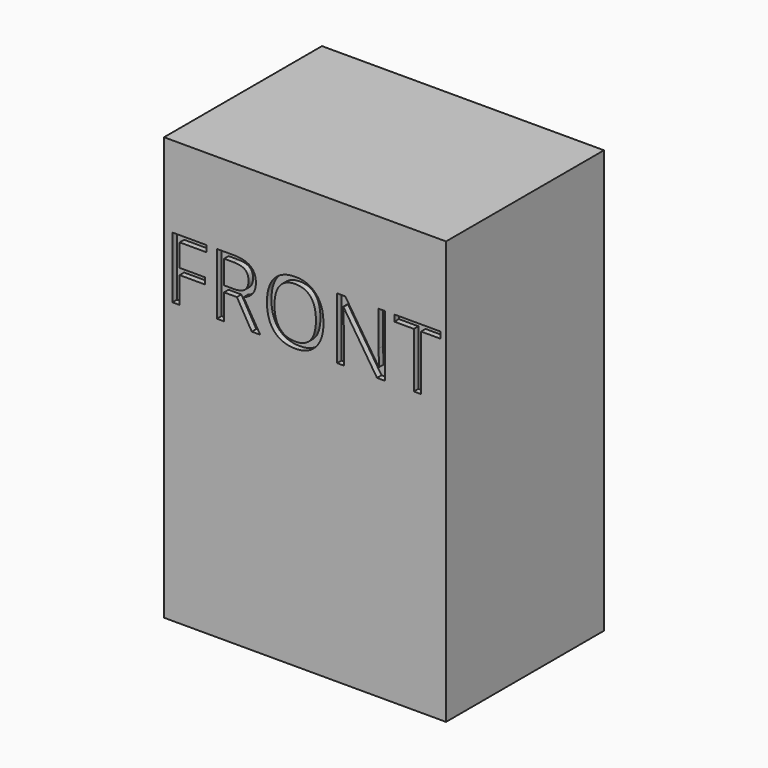
from build123d import *

# Parameters (mm, degrees)
F0_W         = 500
F0_H         = 350
F1_DEPTH     = 750
F2_TEXT_SIZE = 152.6426254532
F3_DEPTH     = 10


# Not quite as in the source:
# - Text() gives the source's letters only with a copy of the font that has no kerning and outlines rounded to 1/6400 em; it was checked with that copy


with BuildPart() as f1:
    # F0 (on Top) → F1 (new body)
    with BuildSketch(Plane.XY):
        with Locations((250, 175)):
            Rectangle(F0_W, F0_H)
    extrude(amount=F1_DEPTH)

    # F2 (on face) → F3 (cut)
    with BuildSketch(Plane.XZ):
        with Locations((0, 497.2021147691)):
            Text('FRONT', F2_TEXT_SIZE, font='Open Sans', text_align=(TextAlign.LEFT, TextAlign.BOTTOM))
    extrude(amount=-F3_DEPTH, mode=Mode.SUBTRACT)


solid = f1.part
